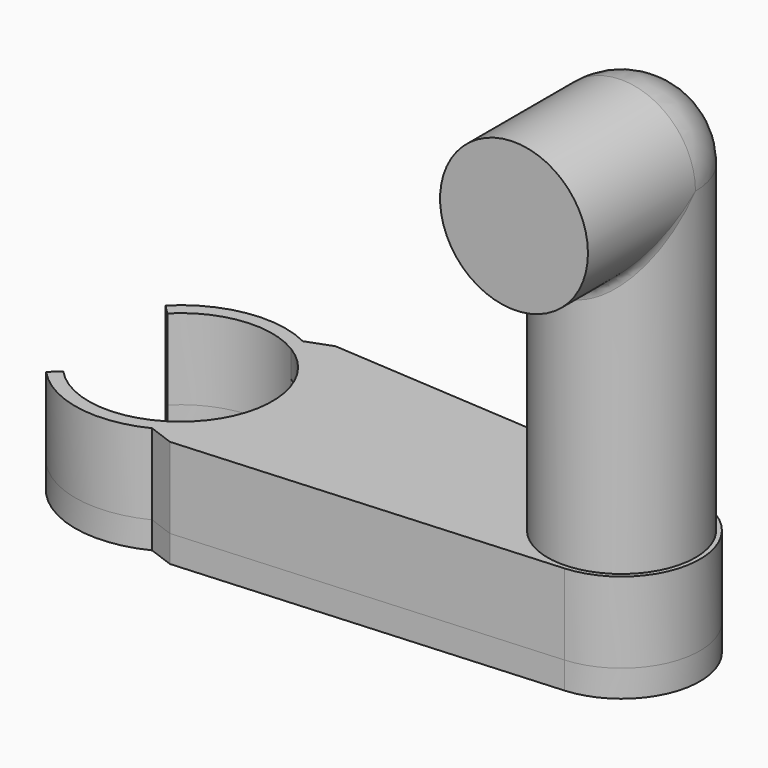
from build123d import *

# Parameters (mm, degrees)
F1_DEPTH = 1
F2_DEPTH = 3
F3_DEPTH = 2
F4_R     = 2.75
F5_DEPTH = 12
F7_ANGLE = 90
F8_R     = 2.75
F9_DEPTH = 5
F10_R    = 0.5


# Not quite as in the source:
# - a feature names something its author has since deleted; it is built from what else it names


with BuildPart() as f1:
    # F0 (on Top) → F1 (new body)
    with BuildSketch(Plane.XY):
        with BuildLine():
            ThreePointArc((1.7856760203, -2.9109424849), (-0.4640879363, -3.3833189899), (-2.5035568051, -2.3225908645))
            Line((-2.5035568051, -2.3225908645), (-2.870109778, -2.6626480921))
            ThreePointArc((-2.870109778, -2.6626480921), (-0.7021528954, -3.8515200001), (1.745866363, -3.5041654702))
            ThreePointArc((1.745866363, -3.5041654702), (2.2390334242, -3.2115345748), (2.6841618804, -2.85))
            Line((2.6841618804, -2.85), (1.7856760203, -2.9109424849))
        make_face()
        with BuildLine():
            ThreePointArc((1.7856760202, 2.910942485), (3.415, 0), (1.7856760203, -2.9109424849))
            Line((1.7856760203, -2.9109424849), (2.6841618804, -2.85))
            ThreePointArc((2.6841618804, -2.85), (3.915, 0), (2.6841618804, 2.85))
            Line((2.6841618803, 2.85), (1.7856760202, 2.910942485))
        make_face()
        with BuildLine():
            ThreePointArc((-2.4179432279, 2.4115919113), (-0.4028376898, 3.391157147), (1.7856760202, 2.910942485))
            Line((1.7856760202, 2.910942485), (2.6841618803, 2.85))
            ThreePointArc((2.6841618804, 2.85), (2.2390334242, 3.2115345748), (1.7458663629, 3.5041654702))
            ThreePointArc((1.7458663629, 3.5041654702), (-0.6323981068, 3.8635861107), (-2.7719612701, 2.7646800388))
            Line((-2.7719612701, 2.7646800388), (-2.4179432279, 2.4115919113))
        make_face()
        with BuildLine():
            Line((16.533754708, -1.9106100332), (2.6841618804, -2.85))
            ThreePointArc((2.6841618804, -2.85), (2.2390334242, -3.2115345748), (1.745866363, -3.5041654702))
            Line((1.745866363, -3.5041654702), (2.6841618804, -3.85))
            Line((2.6841618804, -3.85), (16.6009492353, -2.9083500025))
            ThreePointArc((16.6009492353, -2.9083500025), (19.3191618804, 0), (16.6009492353, 2.9083500025))
            Line((16.6009492353, 2.9083500025), (2.6841618803, 3.85))
            Line((2.6841618803, 3.85), (2.6841618803, 2.85))
            Line((2.6841618803, 2.85), (16.533754708, 1.9106100332))
            ThreePointArc((16.533754708, 1.9106100332), (18.3191618804, 0), (16.533754708, -1.9106100332))
        make_face()
        with BuildLine():
            ThreePointArc((2.6841618804, 2.85), (3.915, 0), (2.6841618804, -2.85))
            Line((2.6841618804, -2.85), (16.533754708, -1.9106100332))
            ThreePointArc((16.533754708, -1.9106100332), (18.3191618804, 0), (16.533754708, 1.9106100332))
            Line((16.533754708, 1.9106100332), (2.6841618803, 2.85))
        make_face()
        with BuildLine():
            ThreePointArc((1.7458663629, 3.5041654702), (2.2390334242, 3.2115345748), (2.6841618804, 2.85))
            Line((2.6841618803, 2.85), (2.6841618803, 3.85))
            Line((2.6841618803, 3.85), (1.7458663629, 3.5041654702))
        make_face()
    extrude(amount=-F1_DEPTH)

    # F0 (on Top) → F2 (join)
    with BuildSketch(Plane.XY):
        with BuildLine():
            ThreePointArc((1.7856760203, -2.9109424849), (-0.4640879363, -3.3833189899), (-2.5035568051, -2.3225908645))
            Line((-2.5035568051, -2.3225908645), (-2.870109778, -2.6626480921))
            ThreePointArc((-2.870109778, -2.6626480921), (-0.7021528954, -3.8515200001), (1.745866363, -3.5041654702))
            ThreePointArc((1.745866363, -3.5041654702), (2.2390334242, -3.2115345748), (2.6841618804, -2.85))
            Line((2.6841618804, -2.85), (1.7856760203, -2.9109424849))
        make_face()
        with BuildLine():
            ThreePointArc((1.7856760202, 2.910942485), (3.415, 0), (1.7856760203, -2.9109424849))
            Line((1.7856760203, -2.9109424849), (2.6841618804, -2.85))
            ThreePointArc((2.6841618804, -2.85), (3.915, 0), (2.6841618804, 2.85))
            Line((2.6841618803, 2.85), (1.7856760202, 2.910942485))
        make_face()
        with BuildLine():
            ThreePointArc((-2.4179432279, 2.4115919113), (-0.4028376898, 3.391157147), (1.7856760202, 2.910942485))
            Line((1.7856760202, 2.910942485), (2.6841618803, 2.85))
            ThreePointArc((2.6841618804, 2.85), (2.2390334242, 3.2115345748), (1.7458663629, 3.5041654702))
            ThreePointArc((1.7458663629, 3.5041654702), (-0.6323981068, 3.8635861107), (-2.7719612701, 2.7646800388))
            Line((-2.7719612701, 2.7646800388), (-2.4179432279, 2.4115919113))
        make_face()
        with BuildLine():
            ThreePointArc((1.7458663629, 3.5041654702), (2.2390334242, 3.2115345748), (2.6841618804, 2.85))
            Line((2.6841618803, 2.85), (2.6841618803, 3.85))
            Line((2.6841618803, 3.85), (1.7458663629, 3.5041654702))
        make_face()
        with BuildLine():
            Line((16.533754708, -1.9106100332), (2.6841618804, -2.85))
            ThreePointArc((2.6841618804, -2.85), (2.2390334242, -3.2115345748), (1.745866363, -3.5041654702))
            Line((1.745866363, -3.5041654702), (2.6841618804, -3.85))
            Line((2.6841618804, -3.85), (16.6009492353, -2.9083500025))
            ThreePointArc((16.6009492353, -2.9083500025), (19.3191618804, 0), (16.6009492353, 2.9083500025))
            Line((16.6009492353, 2.9083500025), (2.6841618803, 3.85))
            Line((2.6841618803, 3.85), (2.6841618803, 2.85))
            Line((2.6841618803, 2.85), (16.533754708, 1.9106100332))
            ThreePointArc((16.533754708, 1.9106100332), (18.3191618804, 0), (16.533754708, -1.9106100332))
        make_face()
        with BuildLine():
            ThreePointArc((2.6841618804, 2.85), (3.915, 0), (2.6841618804, -2.85))
            Line((2.6841618804, -2.85), (16.533754708, -1.9106100332))
            ThreePointArc((16.533754708, -1.9106100332), (18.3191618804, 0), (16.533754708, 1.9106100332))
            Line((16.533754708, 1.9106100332), (2.6841618803, 2.85))
        make_face()
    extrude(amount=F2_DEPTH)

    # F0 (on Top) → F3 (cut)
    with BuildSketch(Plane.XY):
        with BuildLine():
            ThreePointArc((2.6841618804, 2.85), (3.915, 0), (2.6841618804, -2.85))
            Line((2.6841618804, -2.85), (16.533754708, -1.9106100332))
            ThreePointArc((16.533754708, -1.9106100332), (18.3191618804, 0), (16.533754708, 1.9106100332))
            Line((16.533754708, 1.9106100332), (2.6841618803, 2.85))
        make_face()
        with BuildLine():
            ThreePointArc((1.7856760202, 2.910942485), (3.415, 0), (1.7856760203, -2.9109424849))
            Line((1.7856760203, -2.9109424849), (2.6841618804, -2.85))
            ThreePointArc((2.6841618804, -2.85), (3.915, 0), (2.6841618804, 2.85))
            Line((2.6841618803, 2.85), (1.7856760202, 2.910942485))
        make_face()
    extrude(amount=F3_DEPTH, mode=Mode.SUBTRACT)

    # F4 (on face) → F5 (join)
    with BuildSketch(Plane.XY.offset(3)):
        with Locations((16.4041618804, 0)):
            Circle(F4_R)
    extrude(amount=F5_DEPTH)

    # F6 (on face) → F7 (revolve)
    with BuildSketch(Plane.XY.offset(15)):
        with BuildLine():
            Line((13.6541618804, 0), (19.1541618804, 0))
            ThreePointArc((19.1541618804, 0), (16.4041618804, 2.75), (13.6541618804, 0))
        make_face()
    revolve(axis=Axis((16.4041618804, 0, 15), (1, 0, 0)), revolution_arc=F7_ANGLE)

    # F8 (on face) → F9 (join)
    with BuildSketch(Plane.XZ):
        with Locations((16.4041618804, 15)):
            Circle(F8_R)
    extrude(amount=F9_DEPTH)

    # F10
    f10_edges = [f1.edges().sort_by_distance(p)[0] for p in [
        (18.503226, -1.776634, 13.223366),
        (14.305098, -1.776634, 13.223366),
    ]]
    fillet(f10_edges, radius=F10_R)


solid = f1.part
